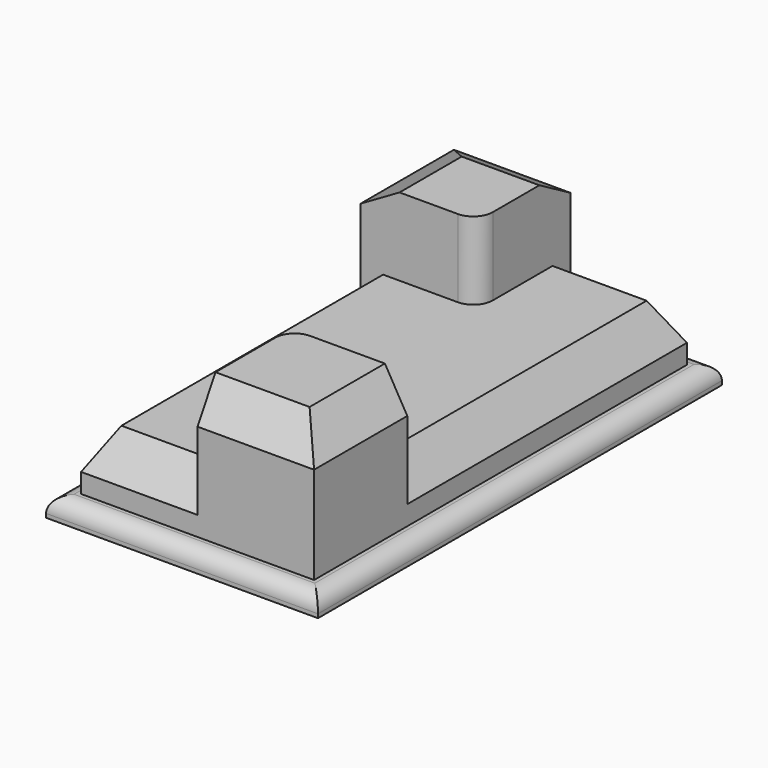
from build123d import *

# Parameters (mm, degrees)
F1_DEPTH    = 25.4
F2_DEPTH    = 50.8
F0_W        = 88.9
F0_H        = 165.1
F3_DEPTH    = 6.35
F4_R        = 5.08
F5_SIZE2    = 7.3323484187
F5_SIZE     = 12.7
F6_C1_SIZE2 = 12.7
F6_C1_SIZE  = 7.3323484187
F6_C2_SIZE2 = 7.3323484187
F6_C2_SIZE  = 12.7
F6_C3_SIZE2 = 12.7
F6_C3_SIZE  = 7.3323484187
F6_C4_SIZE2 = 7.3323484187
F6_C4_SIZE  = 12.7


with BuildPart() as f1:
    # F0 (on Top) → F1 (new body)
    with BuildSketch(Plane.XY):
        with BuildLine():
            Line((-19.5483354544, 60.1456080113), (-51.2983354544, 60.1456080113))
            Line((-51.2983354544, 60.1456080113), (-51.2983354544, -54.1543919887))
            Line((-51.2983354544, -54.1543919887), (-13.1983354544, -54.1543919887))
            Line((-13.1983354544, -54.1543919887), (-13.1983354544, -22.4043919887))
            ThreePointArc((-13.1983354544, -22.4043919887), (-11.3384635149, -17.9142639282), (-6.8483354544, -16.0543919887))
            Line((-6.8483354544, -16.0543919887), (24.9016645456, -16.0543919887))
            Line((24.9016645456, -16.0543919887), (24.9016645456, 98.2456080113))
            Line((24.9016645456, 98.2456080113), (-13.1983354544, 98.2456080113))
            Line((-13.1983354544, 98.2456080113), (-13.1983354544, 66.4956080113))
            ThreePointArc((-13.1983354544, 66.4956080113), (-15.0582073938, 62.0054799508), (-19.5483354544, 60.1456080113))
        make_face()
    extrude(amount=F1_DEPTH)

    # F0 (on Top) → F2 (join)
    with BuildSketch(Plane.XY):
        with BuildLine():
            Line((-13.1983354544, 98.2456080113), (-51.2983354544, 98.2456080113))
            Line((-51.2983354544, 98.2456080113), (-51.2983354544, 60.1456080113))
            Line((-51.2983354544, 60.1456080113), (-19.5483354544, 60.1456080113))
            ThreePointArc((-19.5483354544, 60.1456080113), (-15.0582073938, 62.0054799508), (-13.1983354544, 66.4956080113))
            Line((-13.1983354544, 66.4956080113), (-13.1983354544, 98.2456080113))
        make_face()
        with BuildLine():
            Line((-13.1983354544, -22.4043919887), (-13.1983354544, -54.1543919887))
            Line((-13.1983354544, -54.1543919887), (24.9016645456, -54.1543919887))
            Line((24.9016645456, -54.1543919887), (24.9016645456, -16.0543919887))
            Line((24.9016645456, -16.0543919887), (-6.8483354544, -16.0543919887))
            ThreePointArc((-6.8483354544, -16.0543919887), (-11.3384635149, -17.9142639282), (-13.1983354544, -22.4043919887))
        make_face()
    extrude(amount=F2_DEPTH)

    # F0 (on Top) → F3 (join)
    with BuildSketch(Plane.XY):
        with Locations((-13.1983354544, 22.0456080113)):
            Rectangle(F0_W, F0_H)
        Polygon((-51.2983354544, 60.1456080113), (-51.2983354544, 98.2456080113), (-13.1983354544, 98.2456080113), (24.9016645456, 98.2456080113), (24.9016645456, -16.0543919887), (24.9016645456, -54.1543919887), (-13.1983354544, -54.1543919887), (-51.2983354544, -54.1543919887), align=None, mode=Mode.SUBTRACT)
    extrude(amount=F3_DEPTH)

    # F4
    f4_edges = [f1.edges().sort_by_distance(p)[0] for p in [
        (31.251665, 22.045608, 6.35),
        (-13.198335, -60.504392, 6.35),
        (-57.648335, 22.045608, 6.35),
        (-13.198335, 104.595608, 6.35),
    ]]
    fillet(f4_edges, radius=F4_R)

    # F5
    f5_edges = [f1.edges().sort_by_distance(p)[0] for p in [
        (24.901665, 41.095608, 25.4),
        (5.851665, 98.245608, 25.4),
        (-51.298335, 2.995608, 25.4),
        (-32.248335, -54.154392, 25.4),
    ]]
    chamfer(f5_edges, length=F5_SIZE, length2=F5_SIZE2)

    # F6: chamfer of 12.7 x 7.3323484187 on 4 edges, made by hand

    # F6_c1
    f6_c1_edges = [f1.edges().sort_by_distance(p)[0] for p in [
        (-51.2983354544, 79.1956080113, 50.8),
    ]]
    f6_c1_side = f1.faces().sort_by_distance((-51.2983354544, 79.1956080113, 50.6533530316))[0]
    chamfer(f6_c1_edges, length=F6_C1_SIZE, length2=F6_C1_SIZE2, reference=f6_c1_side)

    # F6_c2
    f6_c2_edges = [f1.edges().sort_by_distance(p)[0] for p in [
        (5.8516645456, -54.1543919887, 50.8),
    ]]
    f6_c2_side = f1.faces().sort_by_distance((5.8516645456, -54.1543919887, 50.6533530316))[0]
    chamfer(f6_c2_edges, length=F6_C2_SIZE, length2=F6_C2_SIZE2, reference=f6_c2_side)

    # F6_c3
    f6_c3_edges = [f1.edges().sort_by_distance(p)[0] for p in [
        (-25.8983354544, 98.2456080113, 50.8),
    ]]
    f6_c3_side = f1.faces().sort_by_distance((-25.8983354544, 98.2456080113, 50.6533530316))[0]
    chamfer(f6_c3_edges, length=F6_C3_SIZE, length2=F6_C3_SIZE2, reference=f6_c3_side)

    # F6_c4
    f6_c4_edges = [f1.edges().sort_by_distance(p)[0] for p in [
        (24.9016645456, -31.4382177794, 50.8),
    ]]
    f6_c4_side = f1.faces().sort_by_distance((24.9016645456, -31.4382177794, 50.6533530316))[0]
    chamfer(f6_c4_edges, length=F6_C4_SIZE, length2=F6_C4_SIZE2, reference=f6_c4_side)


solid = f1.part
